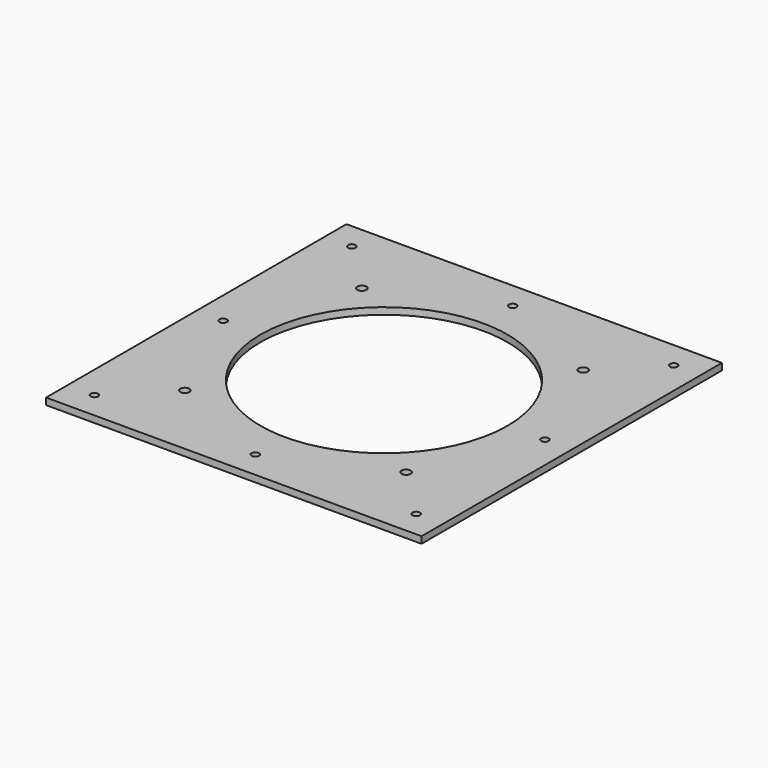
from build123d import *

# Parameters (mm, degrees)
F0_W     = 177.8
F0_H     = 177.8
F0_R     = 1.778
F0_R_2   = 2.159
F0_R_3   = 58.4962
F1_DEPTH = 3.175


# Not quite as in the source:
# - a length typed as a fraction of an inch, garbled in the dataset ("3 / 203.2 mm" for 3/8 in), is restored


with BuildPart() as f1:
    # F0 (on Top) → F1 (new body)
    with BuildSketch(Plane.XY):
        with Locations((88.9, 88.9)):
            Rectangle(F0_W, F0_H)
        with Locations((12.7, 12.7)):
            Circle(F0_R, mode=Mode.SUBTRACT)
        with Locations((36.4998, 36.4998)):
            Circle(F0_R_2, mode=Mode.SUBTRACT)
        with Locations((88.9, 12.7)):
            Circle(F0_R, mode=Mode.SUBTRACT)
        with Locations((165.1, 12.7)):
            Circle(F0_R, mode=Mode.SUBTRACT)
        with Locations((141.3002, 36.4998)):
            Circle(F0_R_2, mode=Mode.SUBTRACT)
        with Locations((12.7, 88.9)):
            Circle(F0_R, mode=Mode.SUBTRACT)
        with Locations((36.4998, 141.3002)):
            Circle(F0_R_2, mode=Mode.SUBTRACT)
        with Locations((12.7, 165.1)):
            Circle(F0_R, mode=Mode.SUBTRACT)
        with Locations((88.9, 88.9)):
            Circle(F0_R_3, mode=Mode.SUBTRACT)
        with Locations((165.1, 88.9)):
            Circle(F0_R, mode=Mode.SUBTRACT)
        with Locations((88.9, 165.1)):
            Circle(F0_R, mode=Mode.SUBTRACT)
        with Locations((141.3002, 141.3002)):
            Circle(F0_R_2, mode=Mode.SUBTRACT)
        with Locations((165.1, 165.1)):
            Circle(F0_R, mode=Mode.SUBTRACT)
    extrude(amount=F1_DEPTH)


solid = f1.part
